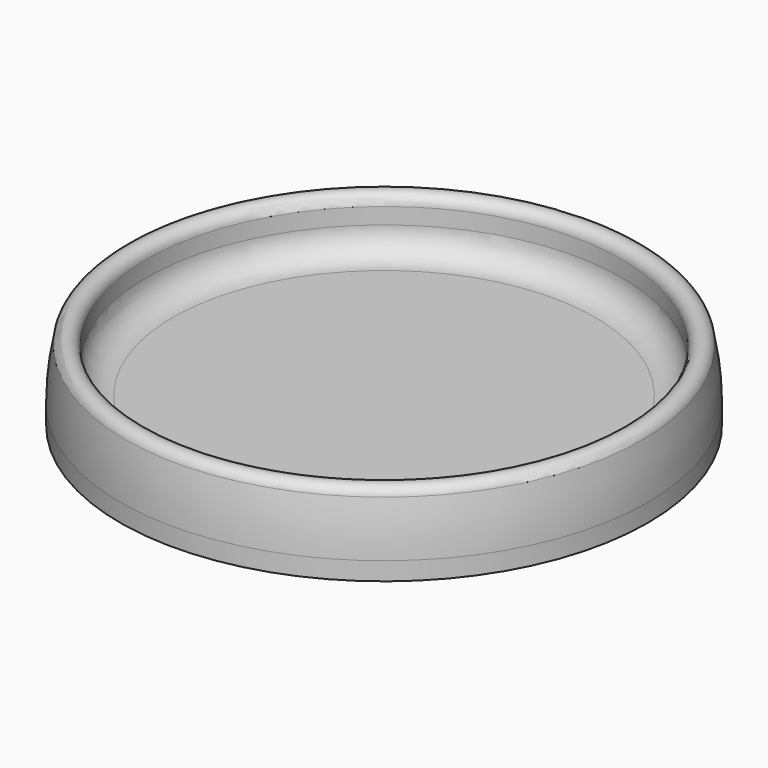
from build123d import *

# Parameters (mm, degrees)
F0_R     = 50
F1_DEPTH = 25
F2_T     = -5
F5_R     = 5


# Not quite as in the source:
# - a fillet or chamfer that OpenCascade refuses, or shapes differently, is made with other operations: its cross-section is extruded or revolved along the edge and cut away or added


with BuildPart() as f1:
    # F0 (on Top) → F1 (new body)
    with BuildSketch(Plane.XY):
        Circle(F0_R)
    extrude(amount=F1_DEPTH)

    # F2
    f2_openings = [f1.faces().sort_by_distance(p)[0] for p in [
        (0, 0, 25),
    ]]
    offset(amount=F2_T, openings=f2_openings)

    # F3: fillet of radius 49 on 1 edges, made by hand

    # F3_s1 → F3_t2 (revolve, cut)
    with BuildSketch(Plane.XZ):
        with BuildLine():
            ThreePointArc((50, 3.4361413472), (48.7336359395, 14.5041131577), (45, 25))
            Line((45, 25), (45.88, 25.4312771731))
            ThreePointArc((45.88, 25.4312771731), (47.5, 25.98), (50, 25.98))
            Line((50, 25.98), (50.98, 25))
            Line((50.98, 25), (50.98, 3.4361413472))
            Line((50.98, 3.4361413472), (50, 3.4361413472))
        make_face()
    revolve(axis=Axis((0, 0, 25), (0, 0, 1)), mode=Mode.SUBTRACT)

    # F4: fillet of radius 2 on 1 edges, made by hand

    # F4_s1 → F4_t2 (revolve, cut)
    with BuildSketch(Plane.XZ):
        with BuildLine():
            ThreePointArc((48.9574468085, 13.4901602258), (46.7937157507, 15.0691253656), (45, 13.0797921083))
            Line((45, 13.0797921083), (45, 25))
            ThreePointArc((45, 25), (47.3374806047, 19.3684321809), (48.9574468085, 13.4901602258))
        make_face()
    revolve(axis=Axis((0, 0, 25), (0, 0, 1)), mode=Mode.SUBTRACT)

    # F5
    f5_edges = [f1.edges().sort_by_distance(p)[0] for p in [
        (-45, 0, 5),
    ]]
    fillet(f5_edges, radius=F5_R)


solid = f1.part
